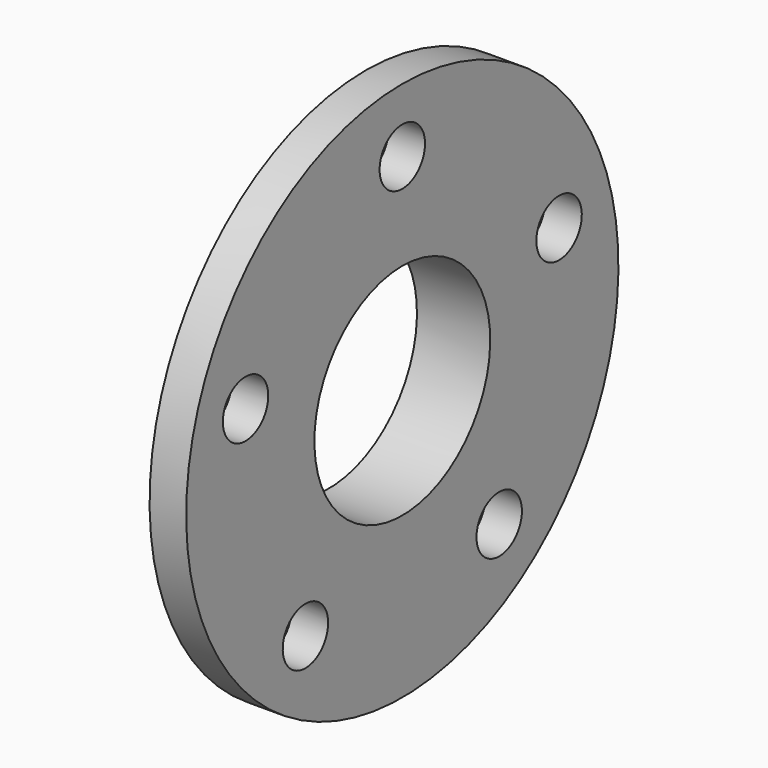
from build123d import *

# Parameters (mm, degrees)
F3_R            = 7.874
F4_DEPTH        = 10.161
F4_COPIES_COUNT = 5


# Not quite as in the source:
# - a pattern or mirror of a feature is missing from the dataset's text; its kind, count and spacing are read off the source's solid


with BuildPart() as f2:
    # F1 (on Front) → F2 (revolve)
    with BuildSketch(Plane.XZ):
        Polygon((0, 36.322), (0, 30.48), (20.32, 30.48), (20.32, 74.93), (10.16, 74.93), (10.16, 36.322), align=None)
    revolve(axis=Axis((6.4773708582, 0, 0), (1, 0, 0)))

    # F3 (on face) → F4 (cut, through all)
    with BuildSketch(Plane(origin=(10.16, 0, 0), x_dir=(0, -1, 0), z_dir=(-1, 0, 0))):
        with Locations((0, 57.15)):
            Circle(F3_R)
    f4 = extrude(amount=-F4_DEPTH, mode=Mode.SUBTRACT)

    # F4_copies: F4 ×5 about axis
    f4_copies_axis = Axis((0, 0, 0), (1, 0, 0))
    for i in range(1, F4_COPIES_COUNT):
        add(f4.rotate(f4_copies_axis, i * 360 / F4_COPIES_COUNT), mode=Mode.SUBTRACT)


solid = f2.part
